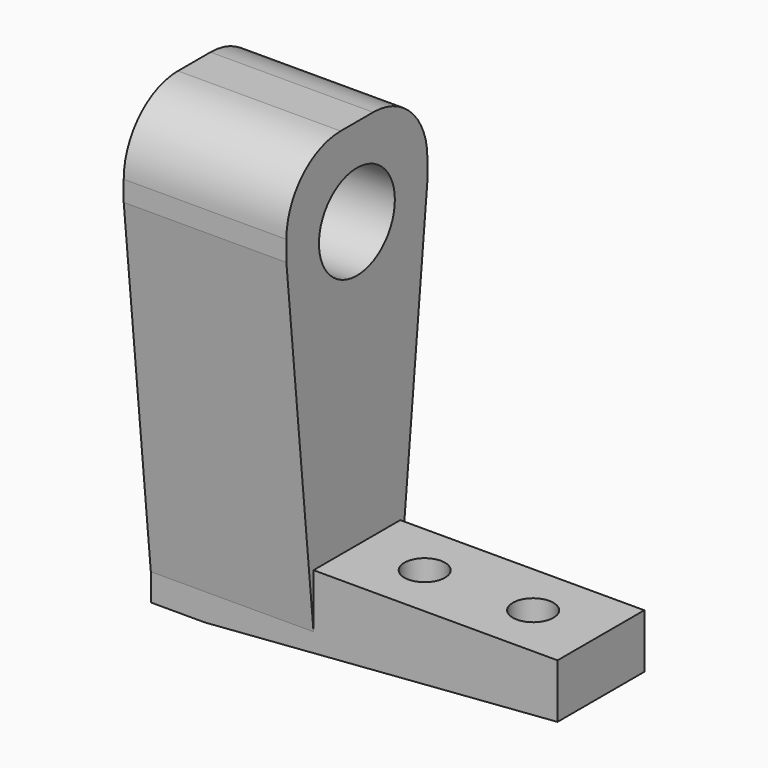
from build123d import *

# Parameters (mm, degrees)
F0_W        = 18
F0_H        = 8
F0_R        = 1.5
F1_DEPTH    = 4
F0_W_2      = 12
F0_H_2      = 2.5
F2_DEPTH    = 31.5
F3_R        = 3.5
F4_DEPTH    = 12.001
F5_R        = 5
F6_DEPTH    = 2
F8_SIZE     = 2.4
F9_T1_DEPTH = 143.1852716253


# Not quite as in the source:
# - a fillet or chamfer that OpenCascade refuses, or shapes differently, is made with other operations: its cross-section is extruded or revolved along the edge and cut away or added


with BuildPart() as f1:
    # F0 (on Top) → F1 (new body)
    with BuildSketch(Plane.XY):
        with Locations((6, 0)):
            Rectangle(F0_W, F0_H)
        with Locations((2, 0)):
            Circle(F0_R, mode=Mode.SUBTRACT)
        with Locations((10, 0)):
            Circle(F0_R, mode=Mode.SUBTRACT)
    extrude(amount=F1_DEPTH)

    # F0 (on Top) → F2 (join)
    with BuildSketch(Plane.XY):
        with Locations((-9, -5.25)):
            Rectangle(F0_W_2, F0_H_2)
        with Locations((-9, 0)):
            Rectangle(F0_W_2, F0_H)
        with Locations((-9, 5.25)):
            Rectangle(F0_W_2, F0_H_2)
    extrude(amount=F2_DEPTH)

    # F3 (on face) → F4 (cut, through all)
    with BuildSketch(Plane.YZ.offset(-3)):
        Polygon((-6.5, 0), (-4, 0), (-6.5, 25), align=None)
        Polygon((6.5, 25), (4, 0), (6.5, 0), align=None)
        with Locations((0, 25)):
            Circle(F3_R)
    extrude(amount=-F4_DEPTH, mode=Mode.SUBTRACT)

    # F5
    f5_edges = [f1.edges().sort_by_distance(p)[0] for p in [
        (-9, 6.5, 31.5),
        (-9, -6.5, 31.5),
    ]]
    fillet(f5_edges, radius=F5_R)

    # F0 (on Top) → F6 (join)
    with BuildSketch(Plane.XY):
        with Locations((6, 0)):
            Rectangle(F0_W, F0_H)
        with Locations((2, 0)):
            Circle(F0_R, mode=Mode.SUBTRACT)
        with Locations((10, 0)):
            Circle(F0_R, mode=Mode.SUBTRACT)
        with Locations((-9, 0)):
            Rectangle(F0_W_2, F0_H)
    extrude(amount=-F6_DEPTH)

    # F7: chamfer of 2 on 1 edges, made by hand

    # F7_s1 → F7_t2 (revolve, cut)
    with BuildSketch(Plane.XZ):
        Polygon((3.5, 0), (5.5, -2), (3.5, -2), align=None)
    revolve(axis=Axis((2, 0, -2), (0, 0, 1)), mode=Mode.SUBTRACT)

    # F8
    f8_edges = [f1.edges().sort_by_distance(p)[0] for p in [
        (8.5, 0, -2),
    ]]
    chamfer(f8_edges, length=F8_SIZE)

    # F9: chamfer of 2 x 26 on 1 edges, made by hand

    # F9_s2 → F9_t1 (cut)
    with BuildSketch(Plane.XZ.offset(-71.5926358126)):
        Polygon((-11, -2), (15, 0), (15, -2), align=None)
    extrude(amount=F9_T1_DEPTH, mode=Mode.SUBTRACT)


solid = f1.part
